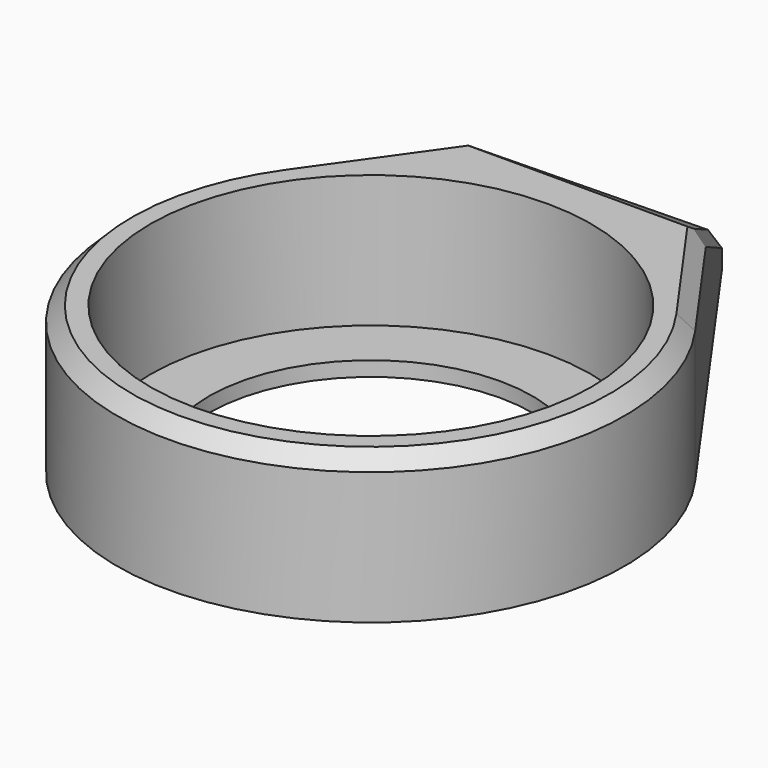
from build123d import *

# Parameters (mm, degrees)
F0_R         = 14.75
F0_R_2       = 11
F1_DEPTH     = 0.5
F3_DEPTH     = 10
F4_R         = 15
F5_DEPTH     = 9
F8_DEPTH     = 12.5
F9_T1_DEPTH  = 11.9079151816
F9_T3_DEPTH  = 20.7352111954
F9_T5_DEPTH  = 20.7352111954
F9_T7_DEPTH  = 11.9079151816
F9_T10_ANGLE = 250.6333606171
F6_R         = 11
F10_DEPTH    = 25


# Not quite as in the source:
# - a fillet or chamfer that OpenCascade refuses, or shapes differently, is made with other operations: its cross-section is extruded or revolved along the edge and cut away or added


with BuildPart() as f1:
    # F0 (on Top) → F1 (new body)
    with BuildSketch(Plane.XY):
        Circle(F0_R)
        Circle(F0_R_2, mode=Mode.SUBTRACT)
    extrude(amount=F1_DEPTH)

    # F2 (on Top) → F3 (join)
    with BuildSketch(Plane.XY):
        with BuildLine():
            Line((0, 29.8393759876), (-14.0754708725, 9.972142183))
            ThreePointArc((-14.0754708725, 9.972142183), (0, -17.25), (14.0754708725, 9.972142183))
            Line((14.0754708725, 9.972142183), (0, 29.8393759876))
        make_face()
    extrude(amount=F3_DEPTH)

    # F4 (on face) → F5 (cut)
    with BuildSketch(Plane.XY.offset(10)):
        Circle(F4_R)
    extrude(amount=-F5_DEPTH, mode=Mode.SUBTRACT)

    # F7 (on Right) → F8 (cut, symmetric)
    with BuildSketch(Plane.YZ):
        Polygon((30.5235402449, 1.681677395), (30.5303540081, 10.6816748157), (16.5303540081, 10.6816748157), align=None)
    extrude(amount=F8_DEPTH, both=True, mode=Mode.SUBTRACT)

    # F9: chamfer of 1 on 5 edges, made by hand

    # F9_s2 → F9_t1 (cut)
    with BuildSketch(Plane(origin=(0, 0, 0), x_dir=(0, 0, 1), z_dir=(-0.578095199, 0.8159693259, 0))):
        Polygon((9, 17.25), (10, 16.25), (10, 17.25), align=None)
    extrude(amount=F9_T1_DEPTH, mode=Mode.SUBTRACT)

    # F9_s4 → F9_t3 (cut)
    with BuildSketch(Plane(origin=(-11.4991327342, 16.2307862132, -10.4391545701), x_dir=(0.8159693259, 0.578095199, 0), z_dir=(0.5118849348, -0.7225149178, 0.4646999108))):
        Polygon((17.25, 12.4696557739), (16.5627169892, 13.4195021219), (17.25, 13.1932286048), align=None)
    extrude(amount=F9_T3_DEPTH, mode=Mode.SUBTRACT)

    # F9_s6 → F9_t5 (cut)
    with BuildSketch(Plane(origin=(0.8850905039, 1.2492868011, -0.8035037766), x_dir=(-0.8159693259, 0.578095199, 0), z_dir=(0.5118849348, 0.7225149178, -0.4646999108))):
        Polygon((17.25, 12.4696557739), (16.5627169892, 13.4195021219), (17.25, 13.1932286048), align=None)
    extrude(amount=F9_T5_DEPTH, mode=Mode.SUBTRACT)

    # F9_s8 → F9_t7 (cut)
    with BuildSketch(Plane(origin=(6.8839085967, 9.7164935241, 0), x_dir=(0, 0, 1), z_dir=(-0.578095199, -0.8159693259, 0))):
        Polygon((9, 17.25), (10, 16.25), (10, 17.25), align=None)
    extrude(amount=F9_T7_DEPTH, mode=Mode.SUBTRACT)

    # F9_s9 → F9_t10 (revolve, cut)
    with BuildSketch(Plane(origin=(0, 0, 0), x_dir=(0, 0, 1), z_dir=(0.578095199, 0.8159693259, 0))):
        Polygon((10, -16.25), (9, -17.25), (10, -17.25), align=None)
    revolve(axis=Axis((0, 0, 10), (0, 0, 1)), revolution_arc=F9_T10_ANGLE, mode=Mode.SUBTRACT)

    # F6 (on face) → F10 (cut)
    with BuildSketch(Plane.XY.offset(1)):
        Circle(F6_R)
    extrude(amount=-F10_DEPTH, mode=Mode.SUBTRACT)


solid = f1.part
